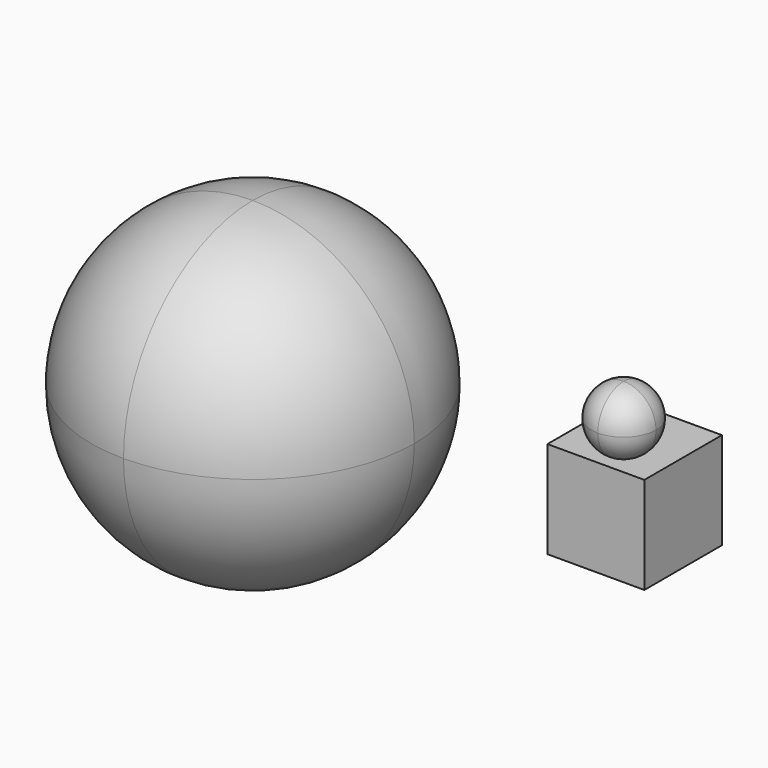
from build123d import *

# Parameters (mm, degrees)
F0_W     = 50
F0_H     = 50
F1_DEPTH = 50
F2_R     = 24.99999
F3_W     = 10
F3_H     = 10
F4_DEPTH = 10
F5_R     = 4.99999
F6_W     = 15
F6_H     = 15
F7_DEPTH = 15


# Not quite as in the source:
# - a fillet or chamfer is up to 0.001 mm smaller than in the source, because OpenCascade refuses the exact size


with BuildPart() as f1:
    # F0 (on Front) → F1 (new body)
    with BuildSketch(Plane.XZ):
        with Locations((7.293150397, 25.0321394791)):
            Rectangle(F0_W, F0_H)
    extrude(amount=F1_DEPTH)

    # F2 (radius 25 in the source; OpenCascade refuses exactly that, so slightly less here)
    f2_edges = [f1.edges().sort_by_distance(p)[0] for p in [
        (-17.70685, -25, 50.032139),
        (32.29315, -25, 50.032139),
        (7.29315, 0, 50.032139),
        (7.29315, -50, 50.032139),
        (-17.70685, 0, 25.032139),
        (7.29315, 0, 0.032139),
        (32.29315, 0, 25.032139),
        (-17.70685, -50, 25.032139),
        (7.29315, -50, 0.032139),
        (32.29315, -50, 25.032139),
        (32.29315, -25, 0.032139),
        (-17.70685, -25, 0.032139),
    ]]
    fillet(f2_edges, radius=F2_R)


with BuildPart() as f4:
    # F3 (on Front) → F4 (new body)
    with BuildSketch(Plane.XZ):
        with Locations((48.6841630191, 25.7099985783)):
            Rectangle(F3_W, F3_H)
    extrude(amount=F4_DEPTH)

    # F5 (radius 5 in the source; OpenCascade refuses exactly that, so slightly less here)
    f5_edges = [f4.edges().sort_by_distance(p)[0] for p in [
        (53.684163, -5, 20.709999),
        (53.684163, -5, 30.709999),
        (53.684163, 0, 25.709999),
        (53.684163, -10, 25.709999),
        (43.684163, -5, 30.709999),
        (48.684163, 0, 30.709999),
        (48.684163, -10, 30.709999),
        (43.684163, -10, 25.709999),
        (48.684163, -10, 20.709999),
        (43.684163, -5, 20.709999),
        (48.684163, 0, 20.709999),
        (43.684163, 0, 25.709999),
    ]]
    fillet(f5_edges, radius=F5_R)


with BuildPart() as f7:
    # F6 (on Top) → F7 (new body)
    with BuildSketch(Plane.XY):
        with Locations((40.3915693331, 7.5)):
            Rectangle(F6_W, F6_H)
    extrude(amount=F7_DEPTH)


solid = Compound([f1.part, f4.part, f7.part])
